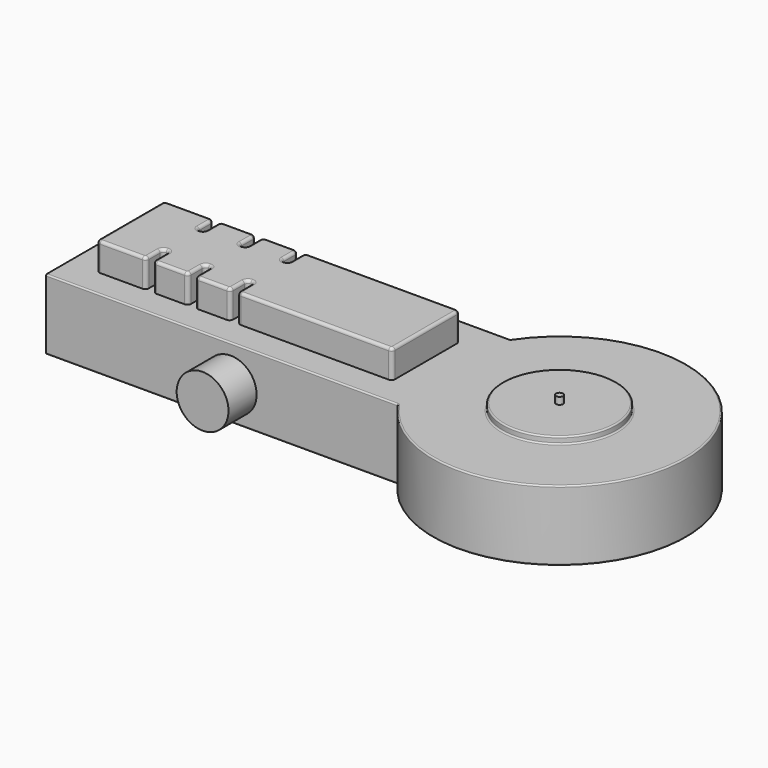
from build123d import *

# Parameters (mm, degrees)
F0_W      = 250
F0_H      = 100
F1_DEPTH  = 50
F3_DEPTH  = 20
F4_R      = 40.3789988007
F5_DEPTH  = 5
F6_R      = 2.5
F7_DEPTH  = 5
F8_R      = 1
F9_R      = 2.49999
F10_R     = 2
F11_R     = 18.4145954801
F12_DEPTH = 25


# Not quite as in the source:
# - a fillet or chamfer is up to 0.001 mm smaller than in the source, because OpenCascade refuses the exact size
# - a feature of the source that left no trace in its solid (it failed there, or was rolled back) is left out


with BuildPart() as f1:
    # F0 (on Top) → F1 (new body)
    with BuildSketch(Plane.XY):
        with Locations((125, 50)):
            Rectangle(F0_W, F0_H)
        with BuildLine():
            Line((250, 100), (250, 0))
            ThreePointArc((250, 0), (415.1387818866, 50), (250, 100))
        make_face()
    extrude(amount=F1_DEPTH)

    # F2 (on face) → F3 (join)
    with BuildSketch(Plane.XY.offset(50)):
        Polygon((55, 80), (20, 80), (20, 20), (55, 20), (55, 35), (60, 35), (60, 20), (85, 20), (85, 35), (90, 35), (90, 20), (115, 20), (115, 35), (120, 35), (120, 20), (230, 20), (230, 80), (120, 80), (120, 65), (115, 65), (115, 80), (90, 80), (90, 65), (85, 65), (85, 80), (60, 80), (60, 65), (55, 65), align=None)
    extrude(amount=F3_DEPTH)

    # F4 (on face) → F5 (join)
    with BuildSketch(Plane.XY.offset(50)):
        with Locations((325, 50)):
            Circle(F4_R)
    extrude(amount=F5_DEPTH)

    # F6 (on face) → F7 (join)
    with BuildSketch(Plane.XY.offset(55)):
        with Locations((325, 50)):
            Circle(F6_R)
    extrude(amount=F7_DEPTH)

    # F8
    f8_edges = [f1.edges().sort_by_distance(p)[0] for p in [
        (250, 0, 25),
        (250, 100, 25),
        (415.138782, 50, 0),
        (415.138782, 50, 50),
        (284.621001, 50, 55),
        (284.621001, 50, 50),
        (125, 100, 0),
        (125, 100, 50),
        (125, 0, 0),
        (125, 0, 50),
    ]]
    fillet(f8_edges, radius=F8_R)

    # F9 (radius 2.5 in the source; OpenCascade refuses exactly that, so slightly less here)
    f9_edges = [f1.edges().sort_by_distance(p)[0] for p in [
        (55, 35, 60),
        (55, 20, 60),
        (60, 35, 60),
        (60, 20, 60),
        (85, 20, 60),
        (90, 35, 60),
        (90, 20, 60),
        (115, 20, 60),
        (120, 35, 60),
        (120, 20, 60),
        (85, 35, 60),
        (115, 35, 60),
        (55, 65, 60),
        (55, 80, 60),
        (85, 65, 60),
        (85, 80, 60),
        (115, 65, 60),
        (115, 80, 60),
        (60, 65, 60),
        (60, 80, 60),
        (90, 65, 60),
        (90, 80, 60),
        (120, 65, 60),
        (120, 80, 60),
        (20, 80, 60),
        (20, 20, 60),
        (230, 80, 60),
        (230, 20, 60),
    ]]
    fillet(f9_edges, radius=F9_R)

    # F10
    f10_edges = [f1.edges().sort_by_distance(p)[0] for p in [
        (175, 80, 70),
        (230, 50, 70),
        (37.5, 80, 70),
        (54.26777, 79.26777, 70),
        (20.73223, 79.26777, 70),
        (55, 72.5, 70),
        (20, 50, 70),
        (55.73223, 65.73223, 70),
        (20.73223, 20.73223, 70),
        (57.5, 65, 70),
        (37.5, 20, 70),
        (59.26777, 65.73223, 70),
        (54.26777, 20.73223, 70),
        (60, 72.5, 70),
        (55, 27.5, 70),
        (60.73223, 79.26777, 70),
        (55.73223, 34.26777, 70),
        (72.5, 80, 70),
        (57.5, 35, 70),
        (84.26777, 79.26777, 70),
        (59.26777, 34.26777, 70),
        (85, 72.5, 70),
        (60, 27.5, 70),
        (85.73223, 65.73223, 70),
        (60.73223, 20.73223, 70),
        (87.5, 65, 70),
        (72.5, 20, 70),
        (89.26777, 65.73223, 70),
        (84.26777, 20.73223, 70),
        (90, 72.5, 70),
        (85, 27.5, 70),
        (90.73223, 79.26777, 70),
        (85.73223, 34.26777, 70),
        (102.5, 80, 70),
        (87.5, 35, 70),
        (114.26777, 79.26777, 70),
        (89.26777, 34.26777, 70),
        (115, 72.5, 70),
        (90, 27.5, 70),
        (115.73223, 65.73223, 70),
        (90.73223, 20.73223, 70),
        (117.5, 65, 70),
        (102.5, 20, 70),
        (119.26777, 65.73223, 70),
        (114.26777, 20.73223, 70),
        (120, 72.5, 70),
        (115, 27.5, 70),
        (120.73223, 79.26777, 70),
        (115.73223, 34.26777, 70),
        (117.5, 35, 70),
        (229.26777, 79.26777, 70),
        (119.26777, 34.26777, 70),
        (120, 27.5, 70),
        (229.26777, 20.73223, 70),
        (120.73223, 20.73223, 70),
        (175, 20, 70),
    ]]
    fillet(f10_edges, radius=F10_R)

    # F11 (on face) → F12 (join)
    with BuildSketch(Plane.XZ):
        with Locations((131.2441378832, 23.4510619193)):
            Circle(F11_R)
    extrude(amount=F12_DEPTH)


solid = f1.part
